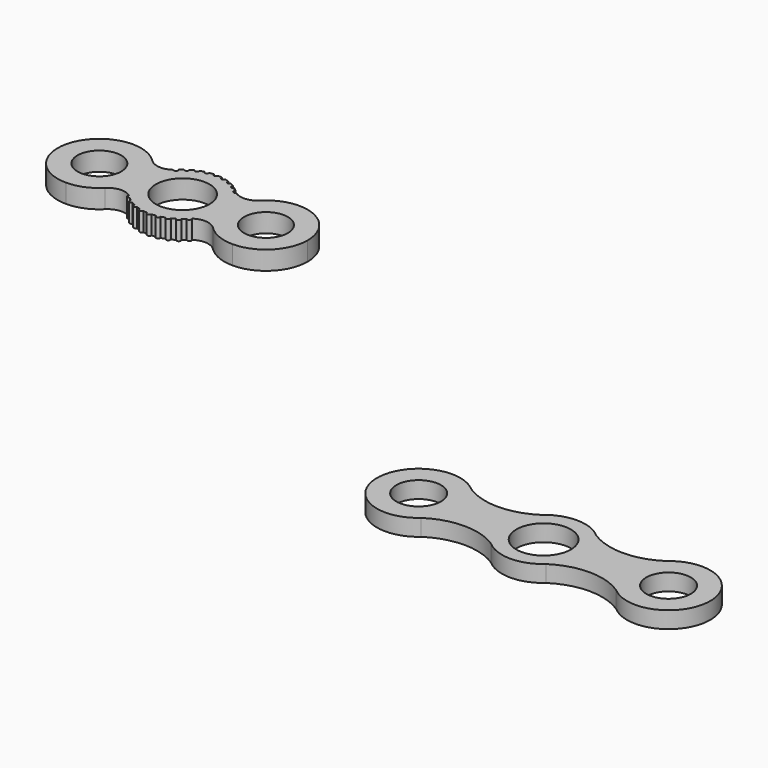
from build123d import *

# Parameters (mm, degrees)
F0_R     = 5.25
F0_R_2   = 6.45
F1_DEPTH = 4.5
F3_R     = 5.35
F3_R_2   = 6.55
F4_DEPTH = 4


with BuildPart() as f1:
    # F0 (on Top) → F1 (new body)
    with BuildSketch(Plane.XY):
        with BuildLine():
            ThreePointArc((12.9289321881, -7.0710678119), (16.1731656763, -9.2387953251), (20, -10))
            ThreePointArc((20, -10), (27.0710678119, -7.0710678119), (30, 0))
            ThreePointArc((30, 0), (23.8268343237, 9.2387953251), (12.9289321881, 7.0710678119))
            ThreePointArc((12.9289321881, 7.0710678119), (10.3293413121, 5.870978103), (7.5723847064, 6.64381593))
            ThreePointArc((7.5723847064, 6.64381593), (6.8533170042, 6.5872309794), (6.8259154618, 7.3080009653))
            ThreePointArc((6.8259154618, 7.3080009653), (6.451016823, 7.6409673438), (6.0598993217, 7.9547231386))
            ThreePointArc((6.0598993217, 7.9547231386), (5.3719769724, 7.835296), (5.235389102, 8.5200176614))
            ThreePointArc((5.235389102, 8.5200176614), (4.8016, 8.7718092455), (4.3557314175, 9.0015334148))
            ThreePointArc((4.3557314175, 9.0015334148), (3.7053332158, 8.7476), (3.4352192125, 9.3914465852))
            ThreePointArc((3.4352192125, 9.3914465852), (2.96, 9.5518793962), (2.4773342567, 9.6882823545))
            ThreePointArc((2.4773342567, 9.6882823545), (1.8904761305, 9.31), (1.4976405546, 9.8872176455))
            ThreePointArc((1.4976405546, 9.8872176455), (1, 9.9498743711), (0.4998437256, 9.9875))
            ThreePointArc((0.4998437256, 9.9875), (0, 9.5), (-0.4998437256, 9.9875))
            ThreePointArc((-0.4998437256, 9.9875), (-1, 9.9498743711), (-1.4976405546, 9.8872176455))
            ThreePointArc((-1.4976405546, 9.8872176455), (-1.8904761305, 9.31), (-2.4773342567, 9.6882823545))
            ThreePointArc((-2.4773342567, 9.6882823545), (-2.96, 9.5518793962), (-3.4352192125, 9.3914465852))
            ThreePointArc((-3.4352192125, 9.3914465852), (-3.7053332158, 8.7476), (-4.3557314175, 9.0015334148))
            ThreePointArc((-4.3557314175, 9.0015334148), (-4.8016, 8.7718092455), (-5.235389102, 8.5200176614))
            ThreePointArc((-5.235389102, 8.5200176614), (-5.3719769724, 7.835296), (-6.0598993217, 7.9547231386))
            ThreePointArc((-6.0598993217, 7.9547231386), (-6.451016823, 7.6409673438), (-6.8259154618, 7.3080009653))
            ThreePointArc((-6.8259154618, 7.3080009653), (-6.8533170042, 6.5872309794), (-7.5723847064, 6.64381593))
            ThreePointArc((-7.5723847064, 6.64381593), (-10.3293413121, 5.870978103), (-12.9289321881, 7.0710678119))
            ThreePointArc((-12.9289321881, 7.0710678119), (-16.1731656763, 9.2387953251), (-20, 10))
            ThreePointArc((-20, 10), (-27.0710678119, 7.0710678119), (-30, 0))
            ThreePointArc((-30, 0), (-27.0710678119, -7.0710678119), (-20, -10))
            ThreePointArc((-20, -10), (-16.1731656763, -9.2387953251), (-12.9289321881, -7.0710678119))
            ThreePointArc((-12.9289321881, -7.0710678119), (-10.3293413121, -5.870978103), (-7.5723847064, -6.64381593))
            ThreePointArc((-7.5723847064, -6.64381593), (-7.0173838095, -6.489948053), (-6.6856824903, -6.9607723876))
            ThreePointArc((-6.6856824903, -6.9607723876), (-6.7220643747, -7.1480108528), (-6.8259154618, -7.3080009653))
            ThreePointArc((-6.8259154618, -7.3080009653), (-6.451016823, -7.6409673438), (-6.0598993217, -7.9547231386))
            ThreePointArc((-6.0598993217, -7.9547231386), (-5.5007537762, -7.7719734941), (-5.1547126026, -8.24768))
            ThreePointArc((-5.1547126026, -8.24768), (-5.1753058075, -8.3896980441), (-5.235389102, -8.5200176614))
            ThreePointArc((-5.235389102, -8.5200176614), (-4.8016, -8.7718092455), (-4.3557314175, -9.0015334148))
            ThreePointArc((-4.3557314175, -9.0015334148), (-3.794734306, -8.7192821202), (-3.4003507535, -9.208))
            ThreePointArc((-3.4003507535, -9.208), (-3.4091452107, -9.3013654902), (-3.4352192125, -9.3914465852))
            ThreePointArc((-3.4352192125, -9.3914465852), (-2.96, -9.5518793962), (-2.4773342567, -9.6882823545))
            ThreePointArc((-2.4773342567, -9.6882823545), (-1.9337596238, -9.3031702046), (-1.4899748742, -9.8))
            ThreePointArc((-1.4899748742, -9.8), (-1.4918949811, -9.8437769355), (-1.4976405546, -9.8872176455))
            ThreePointArc((-1.4976405546, -9.8872176455), (-1, -9.9498743711), (-0.4998437256, -9.9875))
            ThreePointArc((-0.4998437256, -9.9875), (0, -9.5), (0.4998437256, -9.9875))
            ThreePointArc((0.4998437256, -9.9875), (1, -9.9498743711), (1.4976405546, -9.8872176455))
            ThreePointArc((1.4976405546, -9.8872176455), (1.8904761305, -9.31), (2.4773342567, -9.6882823545))
            ThreePointArc((2.4773342567, -9.6882823545), (2.96, -9.5518793962), (3.4352192125, -9.3914465852))
            ThreePointArc((3.4352192125, -9.3914465852), (3.7053332158, -8.7476), (4.3557314175, -9.0015334148))
            ThreePointArc((4.3557314175, -9.0015334148), (4.8016, -8.7718092455), (5.235389102, -8.5200176614))
            ThreePointArc((5.235389102, -8.5200176614), (5.3719769724, -7.835296), (6.0598993217, -7.9547231386))
            ThreePointArc((6.0598993217, -7.9547231386), (6.451016823, -7.6409673438), (6.8259154618, -7.3080009653))
            ThreePointArc((6.8259154618, -7.3080009653), (6.8533170042, -6.5872309794), (7.5723847064, -6.64381593))
            ThreePointArc((7.5723847064, -6.64381593), (10.3293413121, -5.870978103), (12.9289321881, -7.0710678119))
        make_face()
        with Locations((-20, 0)):
            Circle(F0_R, mode=Mode.SUBTRACT)
        Circle(F0_R_2, mode=Mode.SUBTRACT)
        with Locations((20, 0)):
            Circle(F0_R, mode=Mode.SUBTRACT)
        with BuildLine():
            ThreePointArc((7.6856824903, -6.9607723876), (7.6565068249, -6.7924737068), (7.5723847064, -6.64381593))
            ThreePointArc((7.5723847064, -6.64381593), (7.3132200921, -6.8474611419), (7.0710678119, -7.0710678119))
            ThreePointArc((7.0710678119, -7.0710678119), (6.9495014466, -7.1905792286), (6.8259154618, -7.3080009653))
            ThreePointArc((6.8259154618, -7.3080009653), (7.3729209555, -7.4243905032), (7.6856824903, -6.9607723876))
        make_face()
        with BuildLine():
            ThreePointArc((7.0710678119, -7.0710678119), (7.3132200921, -6.8474611419), (7.5723847064, -6.64381593))
            ThreePointArc((7.5723847064, -6.64381593), (6.8533170042, -6.5872309794), (6.8259154618, -7.3080009653))
            ThreePointArc((6.8259154618, -7.3080009653), (6.9495014466, -7.1905792286), (7.0710678119, -7.0710678119))
        make_face()
        with BuildLine():
            ThreePointArc((6.1547126026, -8.24768), (6.1304191085, -8.0937211736), (6.0598993217, -7.9547231386))
            ThreePointArc((6.0598993217, -7.9547231386), (5.6547126026, -8.24768), (5.235389102, -8.5200176614))
            ThreePointArc((5.235389102, -8.5200176614), (5.7967306467, -8.7270867951), (6.1547126026, -8.24768))
        make_face()
        with BuildLine():
            ThreePointArc((5.235389102, -8.5200176614), (5.6547126026, -8.24768), (6.0598993217, -7.9547231386))
            ThreePointArc((6.0598993217, -7.9547231386), (5.3719769724, -7.835296), (5.235389102, -8.5200176614))
        make_face()
        with BuildLine():
            ThreePointArc((4.4003507535, -9.208), (4.3890686332, -9.1023835525), (4.3557314175, -9.0015334148))
            ThreePointArc((4.3557314175, -9.0015334148), (3.9003507535, -9.208), (3.4352192125, -9.3914465852))
            ThreePointArc((3.4352192125, -9.3914465852), (3.9937162437, -9.6992055428), (4.4003507535, -9.208))
        make_face()
        with BuildLine():
            ThreePointArc((3.4352192125, -9.3914465852), (3.9003507535, -9.208), (4.3557314175, -9.0015334148))
            ThreePointArc((4.3557314175, -9.0015334148), (3.7053332158, -8.7476), (3.4352192125, -9.3914465852))
        make_face()
        with BuildLine():
            ThreePointArc((2.4899748742, -9.8), (2.4868046696, -9.7437847496), (2.4773342567, -9.6882823545))
            ThreePointArc((2.4773342567, -9.6882823545), (1.9899748742, -9.8), (1.4976405546, -9.8872176455))
            ThreePointArc((1.4976405546, -9.8872176455), (2.0337518098, -10.2980798931), (2.4899748742, -9.8))
        make_face()
        with BuildLine():
            ThreePointArc((1.4976405546, -9.8872176455), (1.9899748742, -9.8), (2.4773342567, -9.6882823545))
            ThreePointArc((2.4773342567, -9.6882823545), (1.8904761305, -9.31), (1.4976405546, -9.8872176455))
        make_face()
        with BuildLine():
            ThreePointArc((0.5, -10), (0.4999609299, -9.9937495116), (0.4998437256, -9.9875))
            ThreePointArc((0.4998437256, -9.9875), (0, -10), (-0.4998437256, -9.9875))
            ThreePointArc((-0.4998437256, -9.9875), (-0.0062504884, -10.4999609299), (0.5, -10))
        make_face()
        with BuildLine():
            ThreePointArc((-0.4998437256, -9.9875), (0, -10), (0.4998437256, -9.9875))
            ThreePointArc((0.4998437256, -9.9875), (0, -9.5), (-0.4998437256, -9.9875))
        make_face()
        with BuildLine():
            ThreePointArc((-2.4773342567, -9.6882823545), (-2.0894736179, -10.29), (-1.4976405546, -9.8872176455))
            ThreePointArc((-1.4976405546, -9.8872176455), (-1.9899748742, -9.8), (-2.4773342567, -9.6882823545))
        make_face()
        with BuildLine():
            ThreePointArc((-2.4773342567, -9.6882823545), (-1.9899748742, -9.8), (-1.4976405546, -9.8872176455))
            ThreePointArc((-1.4976405546, -9.8872176455), (-1.4918949811, -9.8437769355), (-1.4899748742, -9.8))
            ThreePointArc((-1.4899748742, -9.8), (-1.9337596238, -9.3031702046), (-2.4773342567, -9.6882823545))
        make_face()
        with BuildLine():
            ThreePointArc((-4.3557314175, -9.0015334148), (-4.0953682911, -9.6684), (-3.4352192125, -9.3914465852))
            ThreePointArc((-3.4352192125, -9.3914465852), (-3.9003507535, -9.208), (-4.3557314175, -9.0015334148))
        make_face()
        with BuildLine():
            ThreePointArc((-4.3557314175, -9.0015334148), (-3.9003507535, -9.208), (-3.4352192125, -9.3914465852))
            ThreePointArc((-3.4352192125, -9.3914465852), (-3.4091452107, -9.3013654902), (-3.4003507535, -9.208))
            ThreePointArc((-3.4003507535, -9.208), (-3.794734306, -8.7192821202), (-4.3557314175, -9.0015334148))
        make_face()
        with BuildLine():
            ThreePointArc((-6.0598993217, -7.9547231386), (-5.9374482327, -8.660064), (-5.235389102, -8.5200176614))
            ThreePointArc((-5.235389102, -8.5200176614), (-5.6547126026, -8.24768), (-6.0598993217, -7.9547231386))
        make_face()
        with BuildLine():
            ThreePointArc((-6.0598993217, -7.9547231386), (-5.6547126026, -8.24768), (-5.235389102, -8.5200176614))
            ThreePointArc((-5.235389102, -8.5200176614), (-5.1753058075, -8.3896980441), (-5.1547126026, -8.24768))
            ThreePointArc((-5.1547126026, -8.24768), (-5.5007537762, -7.7719734941), (-6.0598993217, -7.9547231386))
        make_face()
        with BuildLine():
            ThreePointArc((-7.5723847064, -6.64381593), (-7.5180479764, -7.3343137958), (-6.8259154618, -7.3080009653))
            ThreePointArc((-6.8259154618, -7.3080009653), (-6.9495014466, -7.1905792286), (-7.0710678119, -7.0710678119))
            ThreePointArc((-7.0710678119, -7.0710678119), (-7.3132200921, -6.8474611419), (-7.5723847064, -6.64381593))
        make_face()
        with BuildLine():
            ThreePointArc((-7.0710678119, -7.0710678119), (-6.9495014466, -7.1905792286), (-6.8259154618, -7.3080009653))
            ThreePointArc((-6.8259154618, -7.3080009653), (-6.7220643747, -7.1480108528), (-6.6856824903, -6.9607723876))
            ThreePointArc((-6.6856824903, -6.9607723876), (-7.0173838095, -6.489948053), (-7.5723847064, -6.64381593))
            ThreePointArc((-7.5723847064, -6.64381593), (-7.3132200921, -6.8474611419), (-7.0710678119, -7.0710678119))
        make_face()
    extrude(amount=F1_DEPTH)


with BuildPart() as f4:
    # F3 (on Top) → F4 (new body)
    with BuildSketch(Plane.XY):
        with BuildLine():
            ThreePointArc((146.4121165976, -73.9300458055), (154.7977383199, -71.4300458055), (163.1833600423, -73.9300458055))
            ThreePointArc((163.1833600423, -73.9300458055), (179.7977383199, -66.4300458055), (163.1833600423, -58.9300458055))
            ThreePointArc((163.1833600423, -58.9300458055), (154.7977383199, -61.4300458055), (146.4121165976, -58.9300458055))
            ThreePointArc((146.4121165976, -58.9300458055), (139.7977383199, -56.4300458055), (133.1833600423, -58.9300458055))
            ThreePointArc((133.1833600423, -58.9300458055), (124.7977383199, -61.4300458055), (116.4121165976, -58.9300458055))
            ThreePointArc((116.4121165976, -58.9300458055), (99.7977383199, -66.4300458055), (116.4121165976, -73.9300458055))
            ThreePointArc((116.4121165976, -73.9300458055), (124.7977383199, -71.4300458055), (133.1833600423, -73.9300458055))
            ThreePointArc((133.1833600423, -73.9300458055), (139.7977383199, -76.4300458055), (146.4121165976, -73.9300458055))
        make_face()
        with Locations((109.7977383199, -66.4300458055)):
            Circle(F3_R, mode=Mode.SUBTRACT)
        with Locations((139.7977383199, -66.4300458055)):
            Circle(F3_R_2, mode=Mode.SUBTRACT)
        with Locations((169.7977383199, -66.4300458055)):
            Circle(F3_R, mode=Mode.SUBTRACT)
    extrude(amount=F4_DEPTH)


solid = Compound([f1.part, f4.part])
